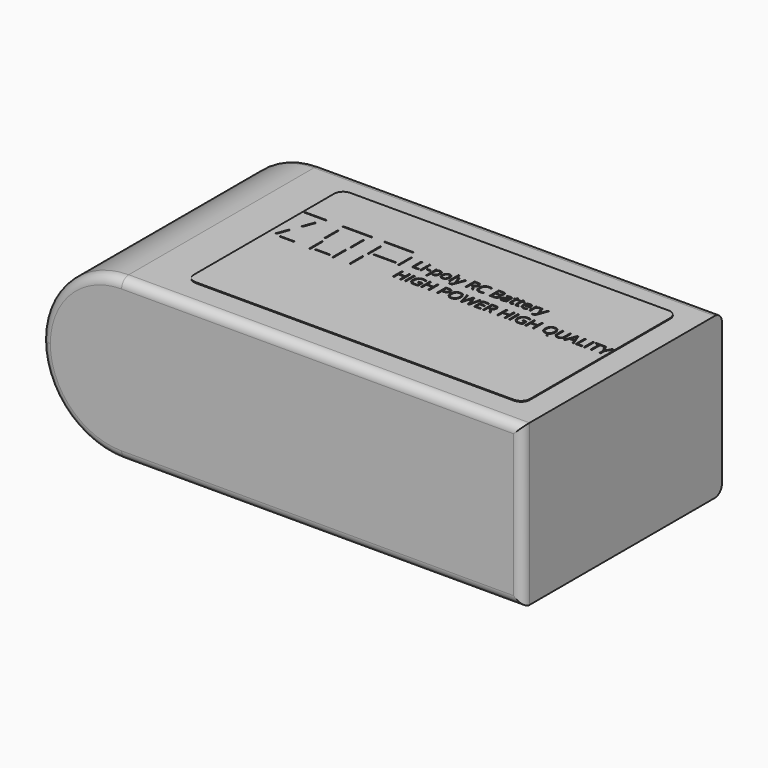
from build123d import *

# Parameters (mm, degrees)
F0_W     = 54
F0_H     = 28
F1_DEPTH = 18
F2_R     = 8.99999
F3_W     = 0.1241319444
F3_H     = 1.8092230903
F3_W_2   = 0.1498046875
F3_H_2   = 1.2889973958
F3_W_3   = 0.1464192708
F3_H_3   = 0.9662543403
F3_W_4   = 0.4327690972
F3_H_4   = 0.1340060764
F3_H_5   = 1.3719401042
F4_DEPTH = 0.1
F5_R     = 1


# Not quite as in the source:
# - a fillet or chamfer is up to 0.001 mm smaller than in the source, because OpenCascade refuses the exact size


with BuildPart() as f1:
    # F0 (on Top) → F1 (new body)
    with BuildSketch(Plane.XY):
        with Locations((-3.3961925656, 5.444671735)):
            Rectangle(F0_W, F0_H)
    extrude(amount=F1_DEPTH)

    # F2 (radius 9 in the source; OpenCascade refuses exactly that, so slightly less here)
    f2_edges = [f1.edges().sort_by_distance(p)[0] for p in [
        (-30.396193, 5.444672, 18),
        (-30.396193, 5.444672, 0),
    ]]
    fillet(f2_edges, radius=F2_R)

    # F3 (on face) → F4 (join)
    with BuildSketch(Plane.XY.offset(18)):
        with BuildLine():
            Line((19.9144558758, 16.5669198185), (-15.8251227587, 16.5669198185))
            ThreePointArc((-15.8251227587, 16.5669198185), (-16.5322295399, 16.2740265997), (-16.8251227587, 15.5669198185))
            Line((-16.8251227587, 15.5669198185), (-16.8251227587, -4.1303987275))
            ThreePointArc((-16.8251227587, -4.1303987275), (-16.5322295399, -4.8375055087), (-15.8251227587, -5.1303987275))
            Line((-15.8251227587, -5.1303987275), (19.9144558758, -5.1303987275))
            ThreePointArc((19.9144558758, -5.1303987275), (20.6215626569, -4.8375055087), (20.9144558758, -4.1303987275))
            Line((20.9144558758, -4.1303987275), (20.9144558758, 15.5669198185))
            ThreePointArc((20.9144558758, 15.5669198185), (20.6215626569, 16.2740265997), (19.9144558758, 16.5669198185))
        make_face()
        Polygon((-15.6610215548, 7.7806734869), (-15.514884402, 7.7806734869), (-15.9953314506, 6.4916760911), (-16.1414686034, 6.4916760911), align=None, mode=Mode.SUBTRACT)
        Polygon((-13.8740857909, 6.2140719244), (-14.6834824923, 6.2140719244), (-14.6905354437, 6.2140719244), (-15.4999321451, 6.2140719244), (-15.4999321451, 6.3294582091), (-14.6905354437, 6.3294582091), (-14.6834824923, 6.3294582091), (-13.8740857909, 6.3294582091), align=None, mode=Mode.SUBTRACT)
        Polygon((-9.8533392631, 6.2140719244), (-10.6627359645, 6.2140719244), (-10.6697889159, 6.2140719244), (-11.4791856173, 6.2140719244), (-11.4791856173, 6.3294582091), (-10.6697889159, 6.3294582091), (-10.6627359645, 6.3294582091), (-9.8533392631, 6.3294582091), align=None, mode=Mode.SUBTRACT)
        with Locations((-11.9723279784, 6.9590046501)):
            Rectangle(F3_W, F3_H, mode=Mode.SUBTRACT)
        Polygon((-14.722696902, 10.2362290425), (-14.5765597492, 10.2362290425), (-15.0570067979, 8.9472316466), (-15.2031439506, 8.9472316466), align=None, mode=Mode.SUBTRACT)
        with Locations((-12.183634402, 9.4145602057)):
            Rectangle(F3_W, F3_H, mode=Mode.SUBTRACT)
        Polygon((-15.0132784992, 11.1251830355), (-15.8156222492, 11.1251830355), (-15.8226752006, 11.1251830355), (-16.632071902, 11.1251830355), (-16.632071902, 11.2405693202), (-15.8226752006, 11.2405693202), (-15.8156222492, 11.2405693202), (-15.0132784992, 11.2405693202), (-15.0062255479, 11.2405693202), (-14.1968288465, 11.2405693202), (-14.1968288465, 11.1251830355), (-15.0062255479, 11.1251830355), align=None, mode=Mode.SUBTRACT)
        Polygon((-10.7084390895, 11.1251830355), (-11.5107828395, 11.1251830355), (-11.5178357909, 11.1251830355), (-12.3272324923, 11.1251830355), (-12.3272324923, 11.2405693202), (-11.5178357909, 11.2405693202), (-11.5107828395, 11.2405693202), (-10.7084390895, 11.2405693202), (-10.7013861381, 11.2405693202), (-9.8990423881, 11.2405693202), (-9.8919894367, 11.2405693202), (-9.0825927354, 11.2405693202), (-9.0825927354, 11.1251830355), (-9.8919894367, 11.1251830355), (-9.8990423881, 11.1251830355), (-10.7013861381, 11.1251830355), align=None, mode=Mode.SUBTRACT)
        with Locations((-9.3590684298, 6.9590046501)):
            Rectangle(F3_W, F3_H, mode=Mode.SUBTRACT)
        with Locations((-7.4262776312, 6.9590046501)):
            Rectangle(F3_W, F3_H, mode=Mode.SUBTRACT)
        Polygon((-5.2677923881, 8.66962748), (-6.0701361381, 8.66962748), (-6.0771890895, 8.66962748), (-6.8865857909, 8.66962748), (-6.8865857909, 8.7850137647), (-6.0771890895, 8.7850137647), (-6.0701361381, 8.7850137647), (-5.2677923881, 8.7850137647), (-5.2607394367, 8.7850137647), (-4.4513427354, 8.7850137647), (-4.4513427354, 8.66962748), (-5.2607394367, 8.66962748), align=None, mode=Mode.SUBTRACT)
        Polygon((-2.0203314506, 7.7806734869), (-2.0203314506, 6.4916760911), (-2.1701361381, 6.4916760911), (-2.1701361381, 7.0982299105), (-2.8491942979, 7.0982299105), (-2.8491942979, 6.4916760911), (-2.9989989854, 6.4916760911), (-2.9989989854, 7.7806734869), (-2.8491942979, 7.7806734869), (-2.8491942979, 7.2322359869), (-2.1701361381, 7.2322359869), (-2.1701361381, 7.7806734869), align=None, mode=Mode.SUBTRACT)
        with Locations((-1.5919351833, 7.136174789)):
            Rectangle(F3_W_2, F3_H_2, mode=Mode.SUBTRACT)
        with BuildLine():
            Line((-0.5964816242, 7.0330606397), (-0.5964816242, 7.1670667161))
            Line((-0.5964816242, 7.1670667161), (-0.158352284, 7.1670667161))
            Line((-0.158352284, 7.1670667161), (-0.158352284, 6.5402003966))
            add(Edge.make_bspline(
                [(-0.158352284, 6.5402003966), (-0.2607611381, 6.5074747022), (-0.366555409, 6.4906886779)],
                knots=[0, 0, 0, 1, 1, 1], degree=2))
            add(Edge.make_bspline(
                [(-0.366555409, 6.4906886779), (-0.4723496798, 6.4739026536), (-0.6117159992, 6.4739026536)],
                knots=[0, 0, 0, 1, 1, 1], degree=2))
            add(Edge.make_bspline(
                [(-0.6117159992, 6.4739026536), (-0.9042724229, 6.4739026536), (-1.067336659, 6.6481105529)],
                knots=[0, 0, 0, 1, 1, 1], degree=2))
            add(Edge.make_bspline(
                [(-1.067336659, 6.6481105529), (-1.2304008951, 6.8223184522), (-1.2304008951, 7.13603373)],
                knots=[0, 0, 0, 1, 1, 1], degree=2))
            add(Edge.make_bspline(
                [(-1.2304008951, 7.13603373), (-1.2304008951, 7.3371839036), (-1.1497151312, 7.4883991813)],
                knots=[0, 0, 0, 1, 1, 1], degree=2))
            add(Edge.make_bspline(
                [(-1.1497151312, 7.4883991813), (-1.0690293673, 7.6396144591), (-0.9173909124, 7.7193128098)],
                knots=[0, 0, 0, 1, 1, 1], degree=2))
            add(Edge.make_bspline(
                [(-0.9173909124, 7.7193128098), (-0.7657524576, 7.7990111605), (-0.5623453395, 7.7990111605)],
                knots=[0, 0, 0, 1, 1, 1], degree=2))
            add(Edge.make_bspline(
                [(-0.5623453395, 7.7990111605), (-0.3558349229, 7.7990111605), (-0.1778184298, 7.7234035216)],
                knots=[0, 0, 0, 1, 1, 1], degree=2))
            Line((-0.1778184298, 7.7234035216), (-0.2359347492, 7.5910901536))
            add(Edge.make_bspline(
                [(-0.2359347492, 7.5910901536), (-0.4105658256, 7.6650050841), (-0.5719373534, 7.6650050841)],
                knots=[0, 0, 0, 1, 1, 1], degree=2))
            add(Edge.make_bspline(
                [(-0.5719373534, 7.6650050841), (-0.8072238117, 7.6650050841), (-0.9395371798, 7.5249334695)],
                knots=[0, 0, 0, 1, 1, 1], degree=2))
            add(Edge.make_bspline(
                [(-0.9395371798, 7.5249334695), (-1.0718505479, 7.384861855), (-1.0718505479, 7.13603373)],
                knots=[0, 0, 0, 1, 1, 1], degree=2))
            add(Edge.make_bspline(
                [(-1.0718505479, 7.13603373), (-1.0718505479, 6.8750745286), (-0.9444742458, 6.740222098)],
                knots=[0, 0, 0, 1, 1, 1], degree=2))
            add(Edge.make_bspline(
                [(-0.9444742458, 6.740222098), (-0.8170979437, 6.6053696675), (-0.5702446451, 6.6053696675)],
                knots=[0, 0, 0, 1, 1, 1], degree=2))
            add(Edge.make_bspline(
                [(-0.5702446451, 6.6053696675), (-0.4362385687, 6.6053696675), (-0.3084390895, 6.6364026536)],
                knots=[0, 0, 0, 1, 1, 1], degree=2))
            Line((-0.3084390895, 6.6364026536), (-0.3084390895, 7.0330606397))
            Line((-0.3084390895, 7.0330606397), (-0.5964816242, 7.0330606397))
        make_face(mode=Mode.SUBTRACT)
        Polygon((1.1295166396, 7.7806734869), (1.1295166396, 6.4916760911), (0.9797119521, 6.4916760911), (0.9797119521, 7.0982299105), (0.3006537924, 7.0982299105), (0.3006537924, 6.4916760911), (0.1508491049, 6.4916760911), (0.1508491049, 7.7806734869), (0.3006537924, 7.7806734869), (0.3006537924, 7.2322359869), (0.9797119521, 7.2322359869), (0.9797119521, 7.7806734869), align=None, mode=Mode.SUBTRACT)
        with Locations((-9.3125189506, 9.4145602057)):
            Rectangle(F3_W, F3_H, mode=Mode.SUBTRACT)
        with Locations((-7.379728152, 9.4145602057)):
            Rectangle(F3_W, F3_H, mode=Mode.SUBTRACT)
        Polygon((-6.0633653048, 11.1251830355), (-6.8657090548, 11.1251830355), (-6.8727620062, 11.1251830355), (-7.6821587076, 11.1251830355), (-7.6821587076, 11.2405693202), (-6.8727620062, 11.2405693202), (-6.8657090548, 11.2405693202), (-6.0633653048, 11.2405693202), (-6.0563123534, 11.2405693202), (-5.2539686034, 11.2405693202), (-5.246915652, 11.2405693202), (-4.4375189506, 11.2405693202), (-4.4375189506, 11.1251830355), (-5.246915652, 11.1251830355), (-5.2539686034, 11.1251830355), (-6.0563123534, 11.1251830355), align=None, mode=Mode.SUBTRACT)
        with Locations((-3.957071902, 9.4145602057)):
            Rectangle(F3_W, F3_H, mode=Mode.SUBTRACT)
        Polygon((-2.0953748534, 8.9472316466), (-2.8139295409, 8.9472316466), (-2.8139295409, 10.2362290425), (-2.6641248534, 10.2362290425), (-2.6641248534, 9.0829304313), (-2.0953748534, 9.0829304313), align=None, mode=Mode.SUBTRACT)
        with Locations((-1.8255289333, 9.4303588168)):
            Rectangle(F3_W_3, F3_H_3, mode=Mode.SUBTRACT)
        with BuildLine():
            add(Edge.make_bspline(
                [(-1.8864664333, 10.10165873), (-1.9111517631, 10.1259208827), (-1.9111517631, 10.1752915425)],
                knots=[0, 0, 0, 1, 1, 1], degree=2))
            add(Edge.make_bspline(
                [(-1.9111517631, 10.1752915425), (-1.9111517631, 10.2255085563), (-1.8864664333, 10.248924355)],
                knots=[0, 0, 0, 1, 1, 1], degree=2))
            add(Edge.make_bspline(
                [(-1.8864664333, 10.248924355), (-1.8617811034, 10.2723401536), (-1.8245415201, 10.2723401536)],
                knots=[0, 0, 0, 1, 1, 1], degree=2))
            add(Edge.make_bspline(
                [(-1.8245415201, 10.2723401536), (-1.7892767631, 10.2723401536), (-1.7637450791, 10.2485011779)],
                knots=[0, 0, 0, 1, 1, 1], degree=2))
            add(Edge.make_bspline(
                [(-1.7637450791, 10.2485011779), (-1.7382133951, 10.2246622022), (-1.7382133951, 10.1752915425)],
                knots=[0, 0, 0, 1, 1, 1], degree=2))
            add(Edge.make_bspline(
                [(-1.7382133951, 10.1752915425), (-1.7382133951, 10.1259208827), (-1.7637450791, 10.10165873)],
                knots=[0, 0, 0, 1, 1, 1], degree=2))
            add(Edge.make_bspline(
                [(-1.7637450791, 10.10165873), (-1.7892767631, 10.0773965772), (-1.8245415201, 10.0773965772)],
                knots=[0, 0, 0, 1, 1, 1], degree=2))
            add(Edge.make_bspline(
                [(-1.8245415201, 10.0773965772), (-1.8617811034, 10.0773965772), (-1.8864664333, 10.10165873)],
                knots=[0, 0, 0, 1, 1, 1], degree=2))
        make_face(mode=Mode.SUBTRACT)
        with BuildLine():
            add(Edge.make_bspline(
                [(-0.1164577527, 9.0613484001), (-0.2226752006, 8.9294582091), (-0.4114121798, 8.9294582091)],
                knots=[0, 0, 0, 1, 1, 1], degree=2))
            add(Edge.make_bspline(
                [(-0.4114121798, 8.9294582091), (-0.5059217284, 8.9294582091), (-0.5839273708, 8.964299789)],
                knots=[0, 0, 0, 1, 1, 1], degree=2))
            add(Edge.make_bspline(
                [(-0.5839273708, 8.964299789), (-0.6619330131, 8.9991413688), (-0.7146890895, 9.0716457091)],
                knots=[0, 0, 0, 1, 1, 1], degree=2))
            Line((-0.7146890895, 9.0716457091), (-0.7254095756, 9.0716457091))
            add(Edge.make_bspline(
                [(-0.7254095756, 9.0716457091), (-0.7146890895, 8.9870102925), (-0.7146890895, 8.9111205355)],
                knots=[0, 0, 0, 1, 1, 1], degree=2))
            Line((-0.7146890895, 8.9111205355), (-0.7146890895, 8.5133340772))
            Line((-0.7146890895, 8.5133340772), (-0.8611083604, 8.5133340772))
            Line((-0.8611083604, 8.5133340772), (-0.8611083604, 9.9134859869))
            Line((-0.8611083604, 9.9134859869), (-0.7420545409, 9.9134859869))
            Line((-0.7420545409, 9.9134859869), (-0.7217420409, 9.7811726188))
            Line((-0.7217420409, 9.7811726188), (-0.7146890895, 9.7811726188))
            add(Edge.make_bspline(
                [(-0.7146890895, 9.7811726188), (-0.6582654784, 9.8607299105), (-0.5833631347, 9.8959946675)],
                knots=[0, 0, 0, 1, 1, 1], degree=2))
            add(Edge.make_bspline(
                [(-0.5833631347, 9.8959946675), (-0.5084607909, 9.9312594244), (-0.4114121798, 9.9312594244)],
                knots=[0, 0, 0, 1, 1, 1], degree=2))
            add(Edge.make_bspline(
                [(-0.4114121798, 9.9312594244), (-0.219289784, 9.9312594244), (-0.1147650444, 9.7997924105)],
                knots=[0, 0, 0, 1, 1, 1], degree=2))
            add(Edge.make_bspline(
                [(-0.1147650444, 9.7997924105), (-0.0102403048, 9.6683253966), (-0.0102403048, 9.43134623)],
                knots=[0, 0, 0, 1, 1, 1], degree=2))
            add(Edge.make_bspline(
                [(-0.0102403048, 9.43134623), (-0.0102403048, 9.1932385911), (-0.1164577527, 9.0613484001)],
                knots=[0, 0, 0, 1, 1, 1], degree=2))
        make_face(mode=Mode.SUBTRACT)
        with Locations((-1.3065727701, 9.4312051709)):
            Rectangle(F3_W_4, F3_H_4, mode=Mode.SUBTRACT)
        with BuildLine():
            add(Edge.make_bspline(
                [(0.9598226292, 9.7962659348), (1.0792996258, 9.6612724452), (1.0792996258, 9.43134623)],
                knots=[0, 0, 0, 1, 1, 1], degree=2))
            add(Edge.make_bspline(
                [(1.0792996258, 9.43134623), (1.0792996258, 9.1949312994), (0.9603868653, 9.0621947543)],
                knots=[0, 0, 0, 1, 1, 1], degree=2))
            add(Edge.make_bspline(
                [(0.9603868653, 9.0621947543), (0.8414741049, 8.9294582091), (0.6315782716, 8.9294582091)],
                knots=[0, 0, 0, 1, 1, 1], degree=2))
            add(Edge.make_bspline(
                [(0.6315782716, 8.9294582091), (0.501803966, 8.9294582091), (0.4013699383, 8.9903957091)],
                knots=[0, 0, 0, 1, 1, 1], degree=2))
            add(Edge.make_bspline(
                [(0.4013699383, 8.9903957091), (0.3009359105, 9.0513332091), (0.2462050077, 9.1650267855)],
                knots=[0, 0, 0, 1, 1, 1], degree=2))
            add(Edge.make_bspline(
                [(0.2462050077, 9.1650267855), (0.1914741049, 9.2787203619), (0.1914741049, 9.43134623)],
                knots=[0, 0, 0, 1, 1, 1], degree=2))
            add(Edge.make_bspline(
                [(0.1914741049, 9.43134623), (0.1914741049, 9.6674790425), (0.3096815702, 9.7993692334)],
                knots=[0, 0, 0, 1, 1, 1], degree=2))
            add(Edge.make_bspline(
                [(0.3096815702, 9.7993692334), (0.4278890355, 9.9312594244), (0.6377848688, 9.9312594244)],
                knots=[0, 0, 0, 1, 1, 1], degree=2))
            add(Edge.make_bspline(
                [(0.6377848688, 9.9312594244), (0.8403456327, 9.9312594244), (0.9598226292, 9.7962659348)],
                knots=[0, 0, 0, 1, 1, 1], degree=2))
        make_face(mode=Mode.SUBTRACT)
        with BuildLine():
            add(Edge.make_bspline(
                [(2.2864827855, 7.7806734869), (2.7694688966, 7.7806734869), (2.7694688966, 7.405174355)],
                knots=[0, 0, 0, 1, 1, 1], degree=2))
            add(Edge.make_bspline(
                [(2.7694688966, 7.405174355), (2.7694688966, 7.2093844244), (2.6358859973, 7.1040133307)],
                knots=[0, 0, 0, 1, 1, 1], degree=2))
            add(Edge.make_bspline(
                [(2.6358859973, 7.1040133307), (2.502303098, 6.9986422369), (2.253757091, 6.9986422369)],
                knots=[0, 0, 0, 1, 1, 1], degree=2))
            Line((2.253757091, 6.9986422369), (2.1019775771, 6.9986422369))
            Line((2.1019775771, 6.9986422369), (2.1019775771, 6.4916760911))
            Line((2.1019775771, 6.4916760911), (1.9521728896, 6.4916760911))
            Line((1.9521728896, 6.4916760911), (1.9521728896, 7.7806734869))
            Line((1.9521728896, 7.7806734869), (2.2864827855, 7.7806734869))
        make_face(mode=Mode.SUBTRACT)
        with BuildLine():
            add(Edge.make_bspline(
                [(4.0020426813, 7.6246622022), (4.158053966, 7.4483384175), (4.158053966, 7.1380085563)],
                knots=[0, 0, 0, 1, 1, 1], degree=2))
            add(Edge.make_bspline(
                [(4.158053966, 7.1380085563), (4.158053966, 6.8285250494), (4.0014784452, 6.6512138515)],
                knots=[0, 0, 0, 1, 1, 1], degree=2))
            add(Edge.make_bspline(
                [(4.0014784452, 6.6512138515), (3.8449029244, 6.4739026536), (3.5664524035, 6.4739026536)],
                knots=[0, 0, 0, 1, 1, 1], degree=2))
            add(Edge.make_bspline(
                [(3.5664524035, 6.4739026536), (3.2817952855, 6.4739026536), (3.127053532, 6.6481105529)],
                knots=[0, 0, 0, 1, 1, 1], degree=2))
            add(Edge.make_bspline(
                [(3.127053532, 6.6481105529), (2.9723117785, 6.8223184522), (2.9723117785, 7.1397012647)],
                knots=[0, 0, 0, 1, 1, 1], degree=2))
            add(Edge.make_bspline(
                [(2.9723117785, 7.1397012647), (2.9723117785, 7.4545450147), (3.1274767091, 7.6277655008)],
                knots=[0, 0, 0, 1, 1, 1], degree=2))
            add(Edge.make_bspline(
                [(3.1274767091, 7.6277655008), (3.2826416396, 7.8009859869), (3.5681451119, 7.8009859869)],
                knots=[0, 0, 0, 1, 1, 1], degree=2))
            add(Edge.make_bspline(
                [(3.5681451119, 7.8009859869), (3.8460313966, 7.8009859869), (4.0020426813, 7.6246622022)],
                knots=[0, 0, 0, 1, 1, 1], degree=2))
        make_face(mode=Mode.SUBTRACT)
        with BuildLine():
            Line((5.915085216, 7.7806734869), (5.5703369521, 6.4916760911))
            Line((5.5703369521, 6.4916760911), (5.422224973, 6.4916760911))
            Line((5.422224973, 6.4916760911), (5.1621121258, 7.354675223))
            add(Edge.make_bspline(
                [(5.1621121258, 7.354675223), (5.1434923341, 7.4122273063), (5.1206407716, 7.4994017855)],
                knots=[0, 0, 0, 1, 1, 1], degree=2))
            add(Edge.make_bspline(
                [(5.1206407716, 7.4994017855), (5.0977892091, 7.5865762647), (5.0969428549, 7.6043497022)],
                knots=[0, 0, 0, 1, 1, 1], degree=2))
            add(Edge.make_bspline(
                [(5.0969428549, 7.6043497022), (5.0774767091, 7.4878349452), (5.0351590008, 7.349597098)],
                knots=[0, 0, 0, 1, 1, 1], degree=2))
            Line((5.0351590008, 7.349597098), (4.7829454591, 6.4916760911))
            Line((4.7829454591, 6.4916760911), (4.6348334799, 6.4916760911))
            Line((4.6348334799, 6.4916760911), (4.2917779244, 7.7806734869))
            Line((4.2917779244, 7.7806734869), (4.4506103896, 7.7806734869))
            Line((4.4506103896, 7.7806734869), (4.6542996258, 6.9845363341))
            add(Edge.make_bspline(
                [(4.6542996258, 6.9845363341), (4.6966173341, 6.8169582091), (4.7160834799, 6.6812594244)],
                knots=[0, 0, 0, 1, 1, 1], degree=2))
            add(Edge.make_bspline(
                [(4.7160834799, 6.6812594244), (4.7397813966, 6.8426309522), (4.7866129938, 6.9969495286)],
                knots=[0, 0, 0, 1, 1, 1], degree=2))
            Line((4.7866129938, 6.9969495286), (5.0173855633, 7.7806734869))
            Line((5.0173855633, 7.7806734869), (5.1762180285, 7.7806734869))
            Line((5.1762180285, 7.7806734869), (5.4185574383, 6.9898965772))
            add(Edge.make_bspline(
                [(5.4185574383, 6.9898965772), (5.4608751466, 6.8530693202), (5.4899333063, 6.6812594244)],
                knots=[0, 0, 0, 1, 1, 1], degree=2))
            add(Edge.make_bspline(
                [(5.4899333063, 6.6812594244), (5.5068603896, 6.8065198411), (5.5534098688, 6.9862290425)],
                knots=[0, 0, 0, 1, 1, 1], degree=2))
            Line((5.5534098688, 6.9862290425), (5.7562527508, 7.7806734869))
            Line((5.7562527508, 7.7806734869), (5.915085216, 7.7806734869))
        make_face(mode=Mode.SUBTRACT)
        Polygon((6.8353543133, 6.6256821675), (6.8353543133, 6.4916760911), (6.1167996258, 6.4916760911), (6.1167996258, 7.7806734869), (6.8353543133, 7.7806734869), (6.8353543133, 7.6475137647), (6.2666043133, 7.6475137647), (6.2666043133, 7.2322359869), (6.8009359105, 7.2322359869), (6.8009359105, 7.0999226188), (6.2666043133, 7.0999226188), (6.2666043133, 6.6256821675), align=None, mode=Mode.SUBTRACT)
        with BuildLine():
            Line((7.539803098, 7.0277003966), (7.270662473, 7.0277003966))
            Line((7.270662473, 7.0277003966), (7.270662473, 6.4916760911))
            Line((7.270662473, 6.4916760911), (7.1208577855, 6.4916760911))
            Line((7.1208577855, 6.4916760911), (7.1208577855, 7.7806734869))
            Line((7.1208577855, 7.7806734869), (7.4743517091, 7.7806734869))
            add(Edge.make_bspline(
                [(7.4743517091, 7.7806734869), (7.7116129938, 7.7806734869), (7.8248833931, 7.689831473)],
                knots=[0, 0, 0, 1, 1, 1], degree=2))
            add(Edge.make_bspline(
                [(7.8248833931, 7.689831473), (7.9381537924, 7.5989894591), (7.9381537924, 7.4164590772)],
                knots=[0, 0, 0, 1, 1, 1], degree=2))
            add(Edge.make_bspline(
                [(7.9381537924, 7.4164590772), (7.9381537924, 7.1608601188), (7.6788872994, 7.0708644591)],
                knots=[0, 0, 0, 1, 1, 1], degree=2))
            Line((7.6788872994, 7.0708644591), (8.0289958063, 6.4916760911))
            Line((8.0289958063, 6.4916760911), (7.8518256674, 6.4916760911))
            Line((7.8518256674, 6.4916760911), (7.539803098, 7.0277003966))
        make_face(mode=Mode.SUBTRACT)
        Polygon((9.6847466744, 7.7806734869), (9.6847466744, 6.4916760911), (9.5349419869, 6.4916760911), (9.5349419869, 7.0982299105), (8.8558838271, 7.0982299105), (8.8558838271, 6.4916760911), (8.7060791396, 6.4916760911), (8.7060791396, 7.7806734869), (8.8558838271, 7.7806734869), (8.8558838271, 7.2322359869), (9.5349419869, 7.2322359869), (9.5349419869, 7.7806734869), align=None, mode=Mode.SUBTRACT)
        with Locations((10.1131429417, 7.136174789)):
            Rectangle(F3_W_2, F3_H_2, mode=Mode.SUBTRACT)
        with BuildLine():
            Line((11.1085965008, 7.0330606397), (11.1085965008, 7.1670667161))
            Line((11.1085965008, 7.1670667161), (11.546725841, 7.1670667161))
            Line((11.546725841, 7.1670667161), (11.546725841, 6.5402003966))
            add(Edge.make_bspline(
                [(11.546725841, 6.5402003966), (11.4443169869, 6.5074747022), (11.338522716, 6.4906886779)],
                knots=[0, 0, 0, 1, 1, 1], degree=2))
            add(Edge.make_bspline(
                [(11.338522716, 6.4906886779), (11.2327284452, 6.4739026536), (11.0933621258, 6.4739026536)],
                knots=[0, 0, 0, 1, 1, 1], degree=2))
            add(Edge.make_bspline(
                [(11.0933621258, 6.4739026536), (10.8008057021, 6.4739026536), (10.637741466, 6.6481105529)],
                knots=[0, 0, 0, 1, 1, 1], degree=2))
            add(Edge.make_bspline(
                [(10.637741466, 6.6481105529), (10.4746772299, 6.8223184522), (10.4746772299, 7.13603373)],
                knots=[0, 0, 0, 1, 1, 1], degree=2))
            add(Edge.make_bspline(
                [(10.4746772299, 7.13603373), (10.4746772299, 7.3371839036), (10.5553629938, 7.4883991813)],
                knots=[0, 0, 0, 1, 1, 1], degree=2))
            add(Edge.make_bspline(
                [(10.5553629938, 7.4883991813), (10.6360487577, 7.6396144591), (10.7876872126, 7.7193128098)],
                knots=[0, 0, 0, 1, 1, 1], degree=2))
            add(Edge.make_bspline(
                [(10.7876872126, 7.7193128098), (10.9393256674, 7.7990111605), (11.1427327855, 7.7990111605)],
                knots=[0, 0, 0, 1, 1, 1], degree=2))
            add(Edge.make_bspline(
                [(11.1427327855, 7.7990111605), (11.3492432021, 7.7990111605), (11.5272596952, 7.7234035216)],
                knots=[0, 0, 0, 1, 1, 1], degree=2))
            Line((11.5272596952, 7.7234035216), (11.4691433758, 7.5910901536))
            add(Edge.make_bspline(
                [(11.4691433758, 7.5910901536), (11.2945122994, 7.6650050841), (11.1331407716, 7.6650050841)],
                knots=[0, 0, 0, 1, 1, 1], degree=2))
            add(Edge.make_bspline(
                [(11.1331407716, 7.6650050841), (10.8978543133, 7.6650050841), (10.7655409452, 7.5249334695)],
                knots=[0, 0, 0, 1, 1, 1], degree=2))
            add(Edge.make_bspline(
                [(10.7655409452, 7.5249334695), (10.6332275771, 7.384861855), (10.6332275771, 7.13603373)],
                knots=[0, 0, 0, 1, 1, 1], degree=2))
            add(Edge.make_bspline(
                [(10.6332275771, 7.13603373), (10.6332275771, 6.8750745286), (10.7606038792, 6.740222098)],
                knots=[0, 0, 0, 1, 1, 1], degree=2))
            add(Edge.make_bspline(
                [(10.7606038792, 6.740222098), (10.8879801813, 6.6053696675), (11.1348334799, 6.6053696675)],
                knots=[0, 0, 0, 1, 1, 1], degree=2))
            add(Edge.make_bspline(
                [(11.1348334799, 6.6053696675), (11.2688395563, 6.6053696675), (11.3966390355, 6.6364026536)],
                knots=[0, 0, 0, 1, 1, 1], degree=2))
            Line((11.3966390355, 6.6364026536), (11.3966390355, 7.0330606397))
            Line((11.3966390355, 7.0330606397), (11.1085965008, 7.0330606397))
        make_face(mode=Mode.SUBTRACT)
        Polygon((12.8345947646, 7.7806734869), (12.8345947646, 6.4916760911), (12.6847900771, 6.4916760911), (12.6847900771, 7.0982299105), (12.0057319174, 7.0982299105), (12.0057319174, 6.4916760911), (11.8559272299, 6.4916760911), (11.8559272299, 7.7806734869), (12.0057319174, 7.7806734869), (12.0057319174, 7.2322359869), (12.6847900771, 7.2322359869), (12.6847900771, 7.7806734869), align=None, mode=Mode.SUBTRACT)
        with BuildLine():
            Line((2.0291911188, 8.9418714036), (1.639303966, 9.9134859869))
            Line((1.639303966, 9.9134859869), (1.796443723, 9.9134859869))
            Line((1.796443723, 9.9134859869), (2.0080322646, 9.3625094244))
            add(Edge.make_bspline(
                [(2.0080322646, 9.3625094244), (2.0774333063, 9.1737724452), (2.0943603896, 9.0899833827)],
                knots=[0, 0, 0, 1, 1, 1], degree=2))
            Line((2.0943603896, 9.0899833827), (2.101413341, 9.0899833827))
            add(Edge.make_bspline(
                [(2.101413341, 9.0899833827), (2.1126980633, 9.1351222716), (2.1493734105, 9.2440198411)],
                knots=[0, 0, 0, 1, 1, 1], degree=2))
            add(Edge.make_bspline(
                [(2.1493734105, 9.2440198411), (2.1860487577, 9.3529174105), (2.3888916396, 9.9134859869)],
                knots=[0, 0, 0, 1, 1, 1], degree=2))
            Line((2.3888916396, 9.9134859869), (2.5457492785, 9.9134859869))
            Line((2.5457492785, 9.9134859869), (2.1304715008, 8.8132255702))
            add(Edge.make_bspline(
                [(2.1304715008, 8.8132255702), (2.0686876466, 8.6501613341), (1.9863091744, 8.5817477057)],
                knots=[0, 0, 0, 1, 1, 1], degree=2))
            add(Edge.make_bspline(
                [(1.9863091744, 8.5817477057), (1.9039307021, 8.5133340772), (1.7840305285, 8.5133340772)],
                knots=[0, 0, 0, 1, 1, 1], degree=2))
            add(Edge.make_bspline(
                [(1.7840305285, 8.5133340772), (1.7168864313, 8.5133340772), (1.6517171605, 8.5285684522)],
                knots=[0, 0, 0, 1, 1, 1], degree=2))
            Line((1.6517171605, 8.5285684522), (1.6517171605, 8.6456474452))
            add(Edge.make_bspline(
                [(1.6517171605, 8.6456474452), (1.700241466, 8.6352090772), (1.7600504938, 8.6352090772)],
                knots=[0, 0, 0, 1, 1, 1], degree=2))
            add(Edge.make_bspline(
                [(1.7600504938, 8.6352090772), (1.9109836535, 8.6352090772), (1.9753065702, 8.8044799105)],
                knots=[0, 0, 0, 1, 1, 1], degree=2))
            Line((1.9753065702, 8.8044799105), (2.0291911188, 8.9418714036))
        make_face(mode=Mode.SUBTRACT)
        with Locations((1.4092366917, 9.6332016987)):
            Rectangle(F3_W_3, F3_H_5, mode=Mode.SUBTRACT)
        with BuildLine():
            Line((3.6127197646, 9.4832559522), (3.3435791396, 9.4832559522))
            Line((3.3435791396, 9.4832559522), (3.3435791396, 8.9472316466))
            Line((3.3435791396, 8.9472316466), (3.1937744521, 8.9472316466))
            Line((3.1937744521, 8.9472316466), (3.1937744521, 10.2362290425))
            Line((3.1937744521, 10.2362290425), (3.5472683758, 10.2362290425))
            add(Edge.make_bspline(
                [(3.5472683758, 10.2362290425), (3.7845296605, 10.2362290425), (3.8978000598, 10.1453870286)],
                knots=[0, 0, 0, 1, 1, 1], degree=2))
            add(Edge.make_bspline(
                [(3.8978000598, 10.1453870286), (4.0110704591, 10.0545450147), (4.0110704591, 9.8720146327)],
                knots=[0, 0, 0, 1, 1, 1], degree=2))
            add(Edge.make_bspline(
                [(4.0110704591, 9.8720146327), (4.0110704591, 9.6164156744), (3.751803966, 9.5264200147)],
                knots=[0, 0, 0, 1, 1, 1], degree=2))
            Line((3.751803966, 9.5264200147), (4.101912473, 8.9472316466))
            Line((4.101912473, 8.9472316466), (3.9247423341, 8.9472316466))
            Line((3.9247423341, 8.9472316466), (3.6127197646, 9.4832559522))
        make_face(mode=Mode.SUBTRACT)
        with BuildLine():
            add(Edge.make_bspline(
                [(5.1544949383, 10.0520059522), (5.0080756674, 10.1205606397), (4.8616563966, 10.1205606397)],
                knots=[0, 0, 0, 1, 1, 1], degree=2))
            add(Edge.make_bspline(
                [(4.8616563966, 10.1205606397), (4.6492215008, 10.1205606397), (4.5262180285, 9.9790784348)],
                knots=[0, 0, 0, 1, 1, 1], degree=2))
            add(Edge.make_bspline(
                [(4.5262180285, 9.9790784348), (4.4032145563, 9.83759623), (4.4032145563, 9.5915892855)],
                knots=[0, 0, 0, 1, 1, 1], degree=2))
            add(Edge.make_bspline(
                [(4.4032145563, 9.5915892855), (4.4032145563, 9.3388115077), (4.5218451987, 9.2007147195)],
                knots=[0, 0, 0, 1, 1, 1], degree=2))
            add(Edge.make_bspline(
                [(4.5218451987, 9.2007147195), (4.640475841, 9.0626179313), (4.8599636883, 9.0626179313)],
                knots=[0, 0, 0, 1, 1, 1], degree=2))
            add(Edge.make_bspline(
                [(4.8599636883, 9.0626179313), (4.9948161188, 9.0626179313), (5.1677544869, 9.1111422369)],
                knots=[0, 0, 0, 1, 1, 1], degree=2))
            Line((5.1677544869, 9.1111422369), (5.1677544869, 8.9799573411))
            add(Edge.make_bspline(
                [(5.1677544869, 8.9799573411), (5.0337484105, 8.9294582091), (4.8371121258, 8.9294582091)],
                knots=[0, 0, 0, 1, 1, 1], degree=2))
            add(Edge.make_bspline(
                [(4.8371121258, 8.9294582091), (4.5524550077, 8.9294582091), (4.3977132542, 9.1023965772)],
                knots=[0, 0, 0, 1, 1, 1], degree=2))
            add(Edge.make_bspline(
                [(4.3977132542, 9.1023965772), (4.2429715008, 9.2753349452), (4.2429715008, 9.5935641119)],
                knots=[0, 0, 0, 1, 1, 1], degree=2))
            add(Edge.make_bspline(
                [(4.2429715008, 9.5935641119), (4.2429715008, 9.7927394591), (4.3174506674, 9.9425441466)],
                knots=[0, 0, 0, 1, 1, 1], degree=2))
            add(Edge.make_bspline(
                [(4.3174506674, 9.9425441466), (4.3919298341, 10.0923488341), (4.5325656848, 10.1734577751)],
                knots=[0, 0, 0, 1, 1, 1], degree=2))
            add(Edge.make_bspline(
                [(4.5325656848, 10.1734577751), (4.6732015355, 10.2545667161), (4.863631223, 10.2545667161)],
                knots=[0, 0, 0, 1, 1, 1], degree=2))
            add(Edge.make_bspline(
                [(4.863631223, 10.2545667161), (5.0661919869, 10.2545667161), (5.2179715008, 10.1806517855)],
                knots=[0, 0, 0, 1, 1, 1], degree=2))
            Line((5.2179715008, 10.1806517855), (5.1544949383, 10.0520059522))
        make_face(mode=Mode.SUBTRACT)
        with BuildLine():
            Line((5.9181885146, 8.9472316466), (5.9181885146, 10.2362290425))
            Line((5.9181885146, 10.2362290425), (6.2824029244, 10.2362290425))
            add(Edge.make_bspline(
                [(6.2824029244, 10.2362290425), (6.5388482369, 10.2362290425), (6.6535292264, 10.1594929313)],
                knots=[0, 0, 0, 1, 1, 1], degree=2))
            add(Edge.make_bspline(
                [(6.6535292264, 10.1594929313), (6.768210216, 10.0827568202), (6.768210216, 9.9171535216)],
                knots=[0, 0, 0, 1, 1, 1], degree=2))
            add(Edge.make_bspline(
                [(6.768210216, 9.9171535216), (6.768210216, 9.802331473), (6.7043104764, 9.7278523063)],
                knots=[0, 0, 0, 1, 1, 1], degree=2))
            add(Edge.make_bspline(
                [(6.7043104764, 9.7278523063), (6.6404107369, 9.6533731397), (6.5176893827, 9.6313679313)],
                knots=[0, 0, 0, 1, 1, 1], degree=2))
            Line((6.5176893827, 9.6313679313), (6.5176893827, 9.6226222716))
            add(Edge.make_bspline(
                [(6.5176893827, 9.6226222716), (6.8113742785, 9.5724052577), (6.8113742785, 9.3139851188)],
                knots=[0, 0, 0, 1, 1, 1], degree=2))
            add(Edge.make_bspline(
                [(6.8113742785, 9.3139851188), (6.8113742785, 9.1413288688), (6.6945774035, 9.0442802577)],
                knots=[0, 0, 0, 1, 1, 1], degree=2))
            add(Edge.make_bspline(
                [(6.6945774035, 9.0442802577), (6.5777805285, 8.9472316466), (6.3678846952, 8.9472316466)],
                knots=[0, 0, 0, 1, 1, 1], degree=2))
            Line((6.3678846952, 8.9472316466), (5.9181885146, 8.9472316466))
        make_face(mode=Mode.SUBTRACT)
        with BuildLine():
            Line((7.7688829591, 8.9472316466), (7.6602675077, 8.9472316466))
            Line((7.6602675077, 8.9472316466), (7.631209348, 9.0849052577))
            Line((7.631209348, 9.0849052577), (7.6241563966, 9.0849052577))
            add(Edge.make_bspline(
                [(7.6241563966, 9.0849052577), (7.5519341744, 8.9940632438), (7.4801351292, 8.9617607265)],
                knots=[0, 0, 0, 1, 1, 1], degree=2))
            add(Edge.make_bspline(
                [(7.4801351292, 8.9617607265), (7.4083360841, 8.9294582091), (7.3005669869, 8.9294582091)],
                knots=[0, 0, 0, 1, 1, 1], degree=2))
            add(Edge.make_bspline(
                [(7.3005669869, 8.9294582091), (7.1569688966, 8.9294582091), (7.0754367785, 9.0036552577)],
                knots=[0, 0, 0, 1, 1, 1], degree=2))
            add(Edge.make_bspline(
                [(7.0754367785, 9.0036552577), (6.9939046605, 9.0778523063), (6.9939046605, 9.2143974452)],
                knots=[0, 0, 0, 1, 1, 1], degree=2))
            add(Edge.make_bspline(
                [(6.9939046605, 9.2143974452), (6.9939046605, 9.5069538688), (7.4619385146, 9.5210597716)],
                knots=[0, 0, 0, 1, 1, 1], degree=2))
            Line((7.4619385146, 9.5210597716), (7.6258491049, 9.5264200147))
            Line((7.6258491049, 9.5264200147), (7.6258491049, 9.5865111605))
            add(Edge.make_bspline(
                [(7.6258491049, 9.5865111605), (7.6258491049, 9.7002047369), (7.5770426813, 9.7543714036)],
                knots=[0, 0, 0, 1, 1, 1], degree=2))
            add(Edge.make_bspline(
                [(7.5770426813, 9.7543714036), (7.5282362577, 9.8085380702), (7.4204671605, 9.8085380702)],
                knots=[0, 0, 0, 1, 1, 1], degree=2))
            add(Edge.make_bspline(
                [(7.4204671605, 9.8085380702), (7.2997206327, 9.8085380702), (7.1473768827, 9.7346231397)],
                knots=[0, 0, 0, 1, 1, 1], degree=2))
            Line((7.1473768827, 9.7346231397), (7.1022379938, 9.8466240077))
            add(Edge.make_bspline(
                [(7.1022379938, 9.8466240077), (7.1736138619, 9.8852741813), (7.2586724556, 9.9072793897)],
                knots=[0, 0, 0, 1, 1, 1], degree=2))
            add(Edge.make_bspline(
                [(7.2586724556, 9.9072793897), (7.3437310494, 9.929284598), (7.4294949383, 9.929284598)],
                knots=[0, 0, 0, 1, 1, 1], degree=2))
            add(Edge.make_bspline(
                [(7.4294949383, 9.929284598), (7.6021511883, 9.929284598), (7.6855170737, 9.8526895459)],
                knots=[0, 0, 0, 1, 1, 1], degree=2))
            add(Edge.make_bspline(
                [(7.6855170737, 9.8526895459), (7.7688829591, 9.7760944938), (7.7688829591, 9.6068236605)],
                knots=[0, 0, 0, 1, 1, 1], degree=2))
            Line((7.7688829591, 9.6068236605), (7.7688829591, 8.9472316466))
        make_face(mode=Mode.SUBTRACT)
        with BuildLine():
            add(Edge.make_bspline(
                [(8.2685140355, 9.0971773932), (8.3099853896, 9.050486855), (8.3822076119, 9.050486855)],
                knots=[0, 0, 0, 1, 1, 1], degree=2))
            add(Edge.make_bspline(
                [(8.3822076119, 9.050486855), (8.4211399035, 9.050486855), (8.4572510146, 9.0561292161)],
                knots=[0, 0, 0, 1, 1, 1], degree=2))
            add(Edge.make_bspline(
                [(8.4572510146, 9.0561292161), (8.4933621258, 9.0617715772), (8.5145209799, 9.0679781744)],
                knots=[0, 0, 0, 1, 1, 1], degree=2))
            Line((8.5145209799, 9.0679781744), (8.5145209799, 8.9559773063))
            add(Edge.make_bspline(
                [(8.5145209799, 8.9559773063), (8.4908230633, 8.9446925841), (8.4445557021, 8.9370753966)],
                knots=[0, 0, 0, 1, 1, 1], degree=2))
            add(Edge.make_bspline(
                [(8.4445557021, 8.9370753966), (8.398288341, 8.9294582091), (8.3610487577, 8.9294582091)],
                knots=[0, 0, 0, 1, 1, 1], degree=2))
            add(Edge.make_bspline(
                [(8.3610487577, 8.9294582091), (8.0809055285, 8.9294582091), (8.0809055285, 9.2248358133)],
                knots=[0, 0, 0, 1, 1, 1], degree=2))
            Line((8.0809055285, 9.2248358133), (8.0809055285, 9.7997924105))
            Line((8.0809055285, 9.7997924105), (7.9423855633, 9.7997924105))
            Line((7.9423855633, 9.7997924105), (7.9423855633, 9.8703219244))
            Line((7.9423855633, 9.8703219244), (8.0809055285, 9.9312594244))
            Line((8.0809055285, 9.9312594244), (8.1424072646, 10.137487723))
            Line((8.1424072646, 10.137487723), (8.2270426813, 10.137487723))
            Line((8.2270426813, 10.137487723), (8.2270426813, 9.9134859869))
            Line((8.2270426813, 9.9134859869), (8.5074680285, 9.9134859869))
            Line((8.5074680285, 9.9134859869), (8.5074680285, 9.7997924105))
            Line((8.5074680285, 9.7997924105), (8.2270426813, 9.7997924105))
            Line((8.2270426813, 9.7997924105), (8.2270426813, 9.2310424105))
            add(Edge.make_bspline(
                [(8.2270426813, 9.2310424105), (8.2270426813, 9.1438679313), (8.2685140355, 9.0971773932)],
                knots=[0, 0, 0, 1, 1, 1], degree=2))
        make_face(mode=Mode.SUBTRACT)
        with BuildLine():
            add(Edge.make_bspline(
                [(8.905818723, 9.0971773932), (8.9472900771, 9.050486855), (9.0195122994, 9.050486855)],
                knots=[0, 0, 0, 1, 1, 1], degree=2))
            add(Edge.make_bspline(
                [(9.0195122994, 9.050486855), (9.058444591, 9.050486855), (9.0945557021, 9.0561292161)],
                knots=[0, 0, 0, 1, 1, 1], degree=2))
            add(Edge.make_bspline(
                [(9.0945557021, 9.0561292161), (9.1306668133, 9.0617715772), (9.1518256674, 9.0679781744)],
                knots=[0, 0, 0, 1, 1, 1], degree=2))
            Line((9.1518256674, 9.0679781744), (9.1518256674, 8.9559773063))
            add(Edge.make_bspline(
                [(9.1518256674, 8.9559773063), (9.1281277508, 8.9446925841), (9.0818603896, 8.9370753966)],
                knots=[0, 0, 0, 1, 1, 1], degree=2))
            add(Edge.make_bspline(
                [(9.0818603896, 8.9370753966), (9.0355930285, 8.9294582091), (8.9983534452, 8.9294582091)],
                knots=[0, 0, 0, 1, 1, 1], degree=2))
            add(Edge.make_bspline(
                [(8.9983534452, 8.9294582091), (8.718210216, 8.9294582091), (8.718210216, 9.2248358133)],
                knots=[0, 0, 0, 1, 1, 1], degree=2))
            Line((8.718210216, 9.2248358133), (8.718210216, 9.7997924105))
            Line((8.718210216, 9.7997924105), (8.5796902508, 9.7997924105))
            Line((8.5796902508, 9.7997924105), (8.5796902508, 9.8703219244))
            Line((8.5796902508, 9.8703219244), (8.718210216, 9.9312594244))
            Line((8.718210216, 9.9312594244), (8.7797119521, 10.137487723))
            Line((8.7797119521, 10.137487723), (8.8643473688, 10.137487723))
            Line((8.8643473688, 10.137487723), (8.8643473688, 9.9134859869))
            Line((8.8643473688, 9.9134859869), (9.144772716, 9.9134859869))
            Line((9.144772716, 9.9134859869), (9.144772716, 9.7997924105))
            Line((9.144772716, 9.7997924105), (8.8643473688, 9.7997924105))
            Line((8.8643473688, 9.7997924105), (8.8643473688, 9.2310424105))
            add(Edge.make_bspline(
                [(8.8643473688, 9.2310424105), (8.8643473688, 9.1438679313), (8.905818723, 9.0971773932)],
                knots=[0, 0, 0, 1, 1, 1], degree=2))
        make_face(mode=Mode.SUBTRACT)
        with BuildLine():
            add(Edge.make_bspline(
                [(9.9200331327, 8.944128348), (9.8509142091, 8.9294582091), (9.7530192438, 8.9294582091)],
                knots=[0, 0, 0, 1, 1, 1], degree=2))
            add(Edge.make_bspline(
                [(9.7530192438, 8.9294582091), (9.5388916396, 8.9294582091), (9.4149007542, 9.0600788688)],
                knots=[0, 0, 0, 1, 1, 1], degree=2))
            add(Edge.make_bspline(
                [(9.4149007542, 9.0600788688), (9.2909098688, 9.1906995286), (9.2909098688, 9.4223184522)],
                knots=[0, 0, 0, 1, 1, 1], degree=2))
            add(Edge.make_bspline(
                [(9.2909098688, 9.4223184522), (9.2909098688, 9.6561943202), (9.4060140355, 9.7937268723)],
                knots=[0, 0, 0, 1, 1, 1], degree=2))
            add(Edge.make_bspline(
                [(9.4060140355, 9.7937268723), (9.5211182021, 9.9312594244), (9.7152154244, 9.9312594244)],
                knots=[0, 0, 0, 1, 1, 1], degree=2))
            add(Edge.make_bspline(
                [(9.7152154244, 9.9312594244), (9.8966173341, 9.9312594244), (10.0024116049, 9.8117824279)],
                knots=[0, 0, 0, 1, 1, 1], degree=2))
            add(Edge.make_bspline(
                [(10.0024116049, 9.8117824279), (10.1082058758, 9.6923054313), (10.1082058758, 9.4965155008)],
                knots=[0, 0, 0, 1, 1, 1], degree=2))
            Line((10.1082058758, 9.4965155008), (10.1082058758, 9.4039807786))
            Line((10.1082058758, 9.4039807786), (9.4426893827, 9.4039807786))
            add(Edge.make_bspline(
                [(9.4426893827, 9.4039807786), (9.4472032716, 9.2338635911), (9.5287353896, 9.1457016987)],
                knots=[0, 0, 0, 1, 1, 1], degree=2))
            add(Edge.make_bspline(
                [(9.5287353896, 9.1457016987), (9.6102675077, 9.0575398063), (9.7583794869, 9.0575398063)],
                knots=[0, 0, 0, 1, 1, 1], degree=2))
            add(Edge.make_bspline(
                [(9.7583794869, 9.0575398063), (9.9143907716, 9.0575398063), (10.0667345216, 9.1227090772)],
                knots=[0, 0, 0, 1, 1, 1], degree=2))
            Line((10.0667345216, 9.1227090772), (10.0667345216, 8.9920884175))
            add(Edge.make_bspline(
                [(10.0667345216, 8.9920884175), (9.9891520563, 8.9587984869), (9.9200331327, 8.944128348)],
                knots=[0, 0, 0, 1, 1, 1], degree=2))
        make_face(mode=Mode.SUBTRACT)
        with BuildLine():
            add(Edge.make_bspline(
                [(10.6320991049, 9.8800549973), (10.7079888619, 9.9312594244), (10.7988308758, 9.9312594244)],
                knots=[0, 0, 0, 1, 1, 1], degree=2))
            add(Edge.make_bspline(
                [(10.7988308758, 9.9312594244), (10.8631537924, 9.9312594244), (10.9142171605, 9.9205389383)],
                knots=[0, 0, 0, 1, 1, 1], degree=2))
            Line((10.9142171605, 9.9205389383), (10.8939046605, 9.7848401536))
            add(Edge.make_bspline(
                [(10.8939046605, 9.7848401536), (10.8340956327, 9.7980997022), (10.7881103896, 9.7980997022)],
                knots=[0, 0, 0, 1, 1, 1], degree=2))
            add(Edge.make_bspline(
                [(10.7881103896, 9.7980997022), (10.6707492785, 9.7980997022), (10.5875244521, 9.7028848584)],
                knots=[0, 0, 0, 1, 1, 1], degree=2))
            add(Edge.make_bspline(
                [(10.5875244521, 9.7028848584), (10.5042996258, 9.6076700147), (10.5042996258, 9.4657646327)],
                knots=[0, 0, 0, 1, 1, 1], degree=2))
            Line((10.5042996258, 9.4657646327), (10.5042996258, 8.9472316466))
            Line((10.5042996258, 8.9472316466), (10.3578803549, 8.9472316466))
            Line((10.3578803549, 8.9472316466), (10.3578803549, 9.9134859869))
            Line((10.3578803549, 9.9134859869), (10.4786268827, 9.9134859869))
            Line((10.4786268827, 9.9134859869), (10.495553966, 9.7346231397))
            Line((10.495553966, 9.7346231397), (10.5026069174, 9.7346231397))
            add(Edge.make_bspline(
                [(10.5026069174, 9.7346231397), (10.556209348, 9.8288505702), (10.6320991049, 9.8800549973)],
                knots=[0, 0, 0, 1, 1, 1], degree=2))
        make_face(mode=Mode.SUBTRACT)
        with BuildLine():
            Line((11.3314697646, 8.9418714036), (10.9415826119, 9.9134859869))
            Line((10.9415826119, 9.9134859869), (11.0987223688, 9.9134859869))
            Line((11.0987223688, 9.9134859869), (11.3103109105, 9.3625094244))
            add(Edge.make_bspline(
                [(11.3103109105, 9.3625094244), (11.3797119521, 9.1737724452), (11.3966390355, 9.0899833827)],
                knots=[0, 0, 0, 1, 1, 1], degree=2))
            Line((11.3966390355, 9.0899833827), (11.4036919869, 9.0899833827))
            add(Edge.make_bspline(
                [(11.4036919869, 9.0899833827), (11.4149767091, 9.1351222716), (11.4516520563, 9.2440198411)],
                knots=[0, 0, 0, 1, 1, 1], degree=2))
            add(Edge.make_bspline(
                [(11.4516520563, 9.2440198411), (11.4883274035, 9.3529174105), (11.6911702855, 9.9134859869)],
                knots=[0, 0, 0, 1, 1, 1], degree=2))
            Line((11.6911702855, 9.9134859869), (11.8480279244, 9.9134859869))
            Line((11.8480279244, 9.9134859869), (11.4327501466, 8.8132255702))
            add(Edge.make_bspline(
                [(11.4327501466, 8.8132255702), (11.3709662924, 8.6501613341), (11.2885878202, 8.5817477057)],
                knots=[0, 0, 0, 1, 1, 1], degree=2))
            add(Edge.make_bspline(
                [(11.2885878202, 8.5817477057), (11.206209348, 8.5133340772), (11.0863091744, 8.5133340772)],
                knots=[0, 0, 0, 1, 1, 1], degree=2))
            add(Edge.make_bspline(
                [(11.0863091744, 8.5133340772), (11.0191650771, 8.5133340772), (10.9539958063, 8.5285684522)],
                knots=[0, 0, 0, 1, 1, 1], degree=2))
            Line((10.9539958063, 8.5285684522), (10.9539958063, 8.6456474452))
            add(Edge.make_bspline(
                [(10.9539958063, 8.6456474452), (11.0025201119, 8.6352090772), (11.0623291396, 8.6352090772)],
                knots=[0, 0, 0, 1, 1, 1], degree=2))
            add(Edge.make_bspline(
                [(11.0623291396, 8.6352090772), (11.2132622994, 8.6352090772), (11.277585216, 8.8044799105)],
                knots=[0, 0, 0, 1, 1, 1], degree=2))
            Line((11.277585216, 8.8044799105), (11.3314697646, 8.9418714036))
        make_face(mode=Mode.SUBTRACT)
        with BuildLine():
            add(Edge.make_bspline(
                [(14.6201199383, 7.6246622022), (14.776131223, 7.4483384175), (14.776131223, 7.1380085563)],
                knots=[0, 0, 0, 1, 1, 1], degree=2))
            add(Edge.make_bspline(
                [(14.776131223, 7.1380085563), (14.776131223, 6.8903089036), (14.6765435494, 6.7262572543)],
                knots=[0, 0, 0, 1, 1, 1], degree=2))
            add(Edge.make_bspline(
                [(14.6765435494, 6.7262572543), (14.5769558758, 6.562205605), (14.395271848, 6.5040892855)],
                knots=[0, 0, 0, 1, 1, 1], degree=2))
            Line((14.395271848, 6.5040892855), (14.7019341744, 6.1847316466))
            Line((14.7019341744, 6.1847316466), (14.4841390355, 6.1847316466))
            Line((14.4841390355, 6.1847316466), (14.233053966, 6.47587748))
            Line((14.233053966, 6.47587748), (14.1845296605, 6.4739026536))
            add(Edge.make_bspline(
                [(14.1845296605, 6.4739026536), (13.8998725424, 6.4739026536), (13.7451307889, 6.6481105529)],
                knots=[0, 0, 0, 1, 1, 1], degree=2))
            add(Edge.make_bspline(
                [(13.7451307889, 6.6481105529), (13.5903890355, 6.8223184522), (13.5903890355, 7.1397012647)],
                knots=[0, 0, 0, 1, 1, 1], degree=2))
            add(Edge.make_bspline(
                [(13.5903890355, 7.1397012647), (13.5903890355, 7.4545450147), (13.745553966, 7.6277655008)],
                knots=[0, 0, 0, 1, 1, 1], degree=2))
            add(Edge.make_bspline(
                [(13.745553966, 7.6277655008), (13.9007188966, 7.8009859869), (14.1862223688, 7.8009859869)],
                knots=[0, 0, 0, 1, 1, 1], degree=2))
            add(Edge.make_bspline(
                [(14.1862223688, 7.8009859869), (14.4641086535, 7.8009859869), (14.6201199383, 7.6246622022)],
                knots=[0, 0, 0, 1, 1, 1], degree=2))
        make_face(mode=Mode.SUBTRACT)
        with BuildLine():
            Line((15.8868300077, 7.7806734869), (16.0366346952, 7.7806734869))
            Line((16.0366346952, 7.7806734869), (16.0366346952, 6.9467325147))
            add(Edge.make_bspline(
                [(16.0366346952, 6.9467325147), (16.0366346952, 6.7261161952), (15.903474973, 6.6000094244)],
                knots=[0, 0, 0, 1, 1, 1], degree=2))
            add(Edge.make_bspline(
                [(15.903474973, 6.6000094244), (15.7703152508, 6.4739026536), (15.5375678549, 6.4739026536)],
                knots=[0, 0, 0, 1, 1, 1], degree=2))
            add(Edge.make_bspline(
                [(15.5375678549, 6.4739026536), (15.3048204591, 6.4739026536), (15.177444157, 6.6009968376)],
                knots=[0, 0, 0, 1, 1, 1], degree=2))
            add(Edge.make_bspline(
                [(15.177444157, 6.6009968376), (15.0500678549, 6.7280910216), (15.0500678549, 6.9501179313)],
                knots=[0, 0, 0, 1, 1, 1], degree=2))
            Line((15.0500678549, 6.9501179313), (15.0500678549, 7.7806734869))
            Line((15.0500678549, 7.7806734869), (15.2001546605, 7.7806734869))
            Line((15.2001546605, 7.7806734869), (15.2001546605, 6.9396795633))
            add(Edge.make_bspline(
                [(15.2001546605, 6.9396795633), (15.2001546605, 6.7783080355), (15.2883165528, 6.6918388515)],
                knots=[0, 0, 0, 1, 1, 1], degree=2))
            add(Edge.make_bspline(
                [(15.2883165528, 6.6918388515), (15.3764784452, 6.6053696675), (15.5474419869, 6.6053696675)],
                knots=[0, 0, 0, 1, 1, 1], degree=2))
            add(Edge.make_bspline(
                [(15.5474419869, 6.6053696675), (15.710506223, 6.6053696675), (15.7986681153, 6.6922620286)],
                knots=[0, 0, 0, 1, 1, 1], degree=2))
            add(Edge.make_bspline(
                [(15.7986681153, 6.6922620286), (15.8868300077, 6.7791543897), (15.8868300077, 6.9413722716)],
                knots=[0, 0, 0, 1, 1, 1], degree=2))
            Line((15.8868300077, 6.9413722716), (15.8868300077, 7.7806734869))
        make_face(mode=Mode.SUBTRACT)
        Polygon((17.3431234105, 6.4916760911), (17.1879584799, 6.4916760911), (17.0274333063, 6.9015936258), (16.5108751466, 6.9015936258), (16.3523247994, 6.4916760911), (16.2005452855, 6.4916760911), (16.7100504938, 7.78603373), (16.8361572646, 7.78603373), align=None, mode=Mode.SUBTRACT)
        Polygon((18.2388482369, 6.4916760911), (17.5202935494, 6.4916760911), (17.5202935494, 7.7806734869), (17.6700982369, 7.7806734869), (17.6700982369, 6.6273748758), (18.2388482369, 6.6273748758), align=None, mode=Mode.SUBTRACT)
        with Locations((18.5323920737, 7.136174789)):
            Rectangle(F3_W_2, F3_H_2, mode=Mode.SUBTRACT)
        Polygon((19.3574463271, 7.6475137647), (19.3574463271, 6.4916760911), (19.2076416396, 6.4916760911), (19.2076416396, 7.6475137647), (18.7994168133, 7.6475137647), (18.7994168133, 7.7806734869), (19.7656711535, 7.7806734869), (19.7656711535, 7.6475137647), align=None, mode=Mode.SUBTRACT)
        Polygon((19.9465088271, 7.7806734869), (20.2878716744, 7.13603373), (20.631491466, 7.7806734869), (20.793709348, 7.7806734869), (20.3634793133, 6.9915892855), (20.3634793133, 6.4916760911), (20.2119819174, 6.4916760911), (20.2119819174, 6.9845363341), (19.7825982369, 7.7806734869), align=None, mode=Mode.SUBTRACT)
        with BuildLine():
            add(Edge.make_bspline(
                [(3.2424398167, 7.5315632438), (3.1308621258, 7.3961465772), (3.1308621258, 7.1380085563)],
                knots=[0, 0, 0, 1, 1, 1], degree=2))
            add(Edge.make_bspline(
                [(3.1308621258, 7.1380085563), (3.1308621258, 6.8762030008), (3.2424398167, 6.7407863341)],
                knots=[0, 0, 0, 1, 1, 1], degree=2))
            add(Edge.make_bspline(
                [(3.2424398167, 6.7407863341), (3.3540175077, 6.6053696675), (3.5664524035, 6.6053696675)],
                knots=[0, 0, 0, 1, 1, 1], degree=2))
            add(Edge.make_bspline(
                [(3.5664524035, 6.6053696675), (3.7805800077, 6.6053696675), (3.8899007542, 6.740222098)],
                knots=[0, 0, 0, 1, 1, 1], degree=2))
            add(Edge.make_bspline(
                [(3.8899007542, 6.740222098), (3.9992215008, 6.8750745286), (3.9992215008, 7.1380085563)],
                knots=[0, 0, 0, 1, 1, 1], degree=2))
            add(Edge.make_bspline(
                [(3.9992215008, 7.1380085563), (3.9992215008, 7.3981214036), (3.8903239313, 7.532550657)],
                knots=[0, 0, 0, 1, 1, 1], degree=2))
            add(Edge.make_bspline(
                [(3.8903239313, 7.532550657), (3.7814263619, 7.6669799105), (3.5681451119, 7.6669799105)],
                knots=[0, 0, 0, 1, 1, 1], degree=2))
            add(Edge.make_bspline(
                [(3.5681451119, 7.6669799105), (3.3540175077, 7.6669799105), (3.2424398167, 7.5315632438)],
                knots=[0, 0, 0, 1, 1, 1], degree=2))
        make_face()
        with BuildLine():
            add(Edge.make_bspline(
                [(13.8605170737, 7.5315632438), (13.7489393827, 7.3961465772), (13.7489393827, 7.1380085563)],
                knots=[0, 0, 0, 1, 1, 1], degree=2))
            add(Edge.make_bspline(
                [(13.7489393827, 7.1380085563), (13.7489393827, 6.8762030008), (13.8605170737, 6.7407863341)],
                knots=[0, 0, 0, 1, 1, 1], degree=2))
            add(Edge.make_bspline(
                [(13.8605170737, 6.7407863341), (13.9720947646, 6.6053696675), (14.1845296605, 6.6053696675)],
                knots=[0, 0, 0, 1, 1, 1], degree=2))
            add(Edge.make_bspline(
                [(14.1845296605, 6.6053696675), (14.3986572646, 6.6053696675), (14.5079780112, 6.740222098)],
                knots=[0, 0, 0, 1, 1, 1], degree=2))
            add(Edge.make_bspline(
                [(14.5079780112, 6.740222098), (14.6172987577, 6.8750745286), (14.6172987577, 7.1380085563)],
                knots=[0, 0, 0, 1, 1, 1], degree=2))
            add(Edge.make_bspline(
                [(14.6172987577, 7.1380085563), (14.6172987577, 7.3981214036), (14.5084011883, 7.532550657)],
                knots=[0, 0, 0, 1, 1, 1], degree=2))
            add(Edge.make_bspline(
                [(14.5084011883, 7.532550657), (14.3995036188, 7.6669799105), (14.1862223688, 7.6669799105)],
                knots=[0, 0, 0, 1, 1, 1], degree=2))
            add(Edge.make_bspline(
                [(14.1862223688, 7.6669799105), (13.9720947646, 7.6669799105), (13.8605170737, 7.5315632438)],
                knots=[0, 0, 0, 1, 1, 1], degree=2))
        make_face()
        with BuildLine():
            add(Edge.make_bspline(
                [(0.4164632542, 9.7124768723), (0.3432536188, 9.6181083827), (0.3432536188, 9.43134623)],
                knots=[0, 0, 0, 1, 1, 1], degree=2))
            add(Edge.make_bspline(
                [(0.3432536188, 9.43134623), (0.3432536188, 9.2459946675), (0.4173096084, 9.1490871154)],
                knots=[0, 0, 0, 1, 1, 1], degree=2))
            add(Edge.make_bspline(
                [(0.4173096084, 9.1490871154), (0.491365598, 9.0521795633), (0.6349636883, 9.0521795633)],
                knots=[0, 0, 0, 1, 1, 1], degree=2))
            add(Edge.make_bspline(
                [(0.6349636883, 9.0521795633), (0.7788438966, 9.0521795633), (0.8533230633, 9.1486639383)],
                knots=[0, 0, 0, 1, 1, 1], degree=2))
            add(Edge.make_bspline(
                [(0.8533230633, 9.1486639383), (0.9278022299, 9.2451483133), (0.9278022299, 9.43134623)],
                knots=[0, 0, 0, 1, 1, 1], degree=2))
            add(Edge.make_bspline(
                [(0.9278022299, 9.43134623), (0.9278022299, 9.6155693202), (0.8533230633, 9.7112073411)],
                knots=[0, 0, 0, 1, 1, 1], degree=2))
            add(Edge.make_bspline(
                [(0.8533230633, 9.7112073411), (0.7788438966, 9.8068453619), (0.6332709799, 9.8068453619)],
                knots=[0, 0, 0, 1, 1, 1], degree=2))
            add(Edge.make_bspline(
                [(0.6332709799, 9.8068453619), (0.4896728896, 9.8068453619), (0.4164632542, 9.7124768723)],
                knots=[0, 0, 0, 1, 1, 1], degree=2))
        make_face()
        with BuildLine():
            add(Edge.make_bspline(
                [(-0.2329725097, 9.7103609869), (-0.3039252006, 9.8068453619), (-0.432571034, 9.8068453619)],
                knots=[0, 0, 0, 1, 1, 1], degree=2))
            add(Edge.make_bspline(
                [(-0.432571034, 9.8068453619), (-0.5806830131, 9.8068453619), (-0.6468396972, 9.7248900668)],
                knots=[0, 0, 0, 1, 1, 1], degree=2))
            add(Edge.make_bspline(
                [(-0.6468396972, 9.7248900668), (-0.7129963812, 9.6429347716), (-0.7146890895, 9.4637898063)],
                knots=[0, 0, 0, 1, 1, 1], degree=2))
            Line((-0.7146890895, 9.4637898063), (-0.7146890895, 9.43134623))
            add(Edge.make_bspline(
                [(-0.7146890895, 9.43134623), (-0.7146890895, 9.2276569938), (-0.6468396972, 9.1399182786)],
                knots=[0, 0, 0, 1, 1, 1], degree=2))
            add(Edge.make_bspline(
                [(-0.6468396972, 9.1399182786), (-0.5789903048, 9.0521795633), (-0.4291856173, 9.0521795633)],
                knots=[0, 0, 0, 1, 1, 1], degree=2))
            add(Edge.make_bspline(
                [(-0.4291856173, 9.0521795633), (-0.3039252006, 9.0521795633), (-0.2329725097, 9.1536010043)],
                knots=[0, 0, 0, 1, 1, 1], degree=2))
            add(Edge.make_bspline(
                [(-0.2329725097, 9.1536010043), (-0.1620198187, 9.2550224452), (-0.1620198187, 9.4330389383)],
                knots=[0, 0, 0, 1, 1, 1], degree=2))
            add(Edge.make_bspline(
                [(-0.1620198187, 9.4330389383), (-0.1620198187, 9.6138766119), (-0.2329725097, 9.7103609869)],
                knots=[0, 0, 0, 1, 1, 1], degree=2))
        make_face()
        with BuildLine():
            Line((6.3247206327, 9.5574530008), (6.0679932021, 9.5574530008))
            Line((6.0679932021, 9.5574530008), (6.0679932021, 9.0750311258))
            Line((6.0679932021, 9.0750311258), (6.3371338271, 9.0750311258))
            add(Edge.make_bspline(
                [(6.3371338271, 9.0750311258), (6.4931451119, 9.0750311258), (6.5719971084, 9.1354043897)],
                knots=[0, 0, 0, 1, 1, 1], degree=2))
            add(Edge.make_bspline(
                [(6.5719971084, 9.1354043897), (6.6508491049, 9.1957776536), (6.6508491049, 9.324705605)],
                knots=[0, 0, 0, 1, 1, 1], degree=2))
            add(Edge.make_bspline(
                [(6.6508491049, 9.324705605), (6.6508491049, 9.4446057786), (6.570163341, 9.5010293897)],
                knots=[0, 0, 0, 1, 1, 1], degree=2))
            add(Edge.make_bspline(
                [(6.570163341, 9.5010293897), (6.4894775771, 9.5574530008), (6.3247206327, 9.5574530008)],
                knots=[0, 0, 0, 1, 1, 1], degree=2))
        make_face()
        with BuildLine():
            Line((2.1019775771, 7.6508991813), (2.1019775771, 7.1272880702))
            Line((2.1019775771, 7.1272880702), (2.2371121258, 7.1272880702))
            add(Edge.make_bspline(
                [(2.2371121258, 7.1272880702), (2.436287473, 7.1272880702), (2.5252957195, 7.1916109869)],
                knots=[0, 0, 0, 1, 1, 1], degree=2))
            add(Edge.make_bspline(
                [(2.5252957195, 7.1916109869), (2.614303966, 7.2559339036), (2.614303966, 7.3981214036)],
                knots=[0, 0, 0, 1, 1, 1], degree=2))
            add(Edge.make_bspline(
                [(2.614303966, 7.3981214036), (2.614303966, 7.5259208827), (2.5305149035, 7.588410032)],
                knots=[0, 0, 0, 1, 1, 1], degree=2))
            add(Edge.make_bspline(
                [(2.5305149035, 7.588410032), (2.446725841, 7.6508991813), (2.2695557021, 7.6508991813)],
                knots=[0, 0, 0, 1, 1, 1], degree=2))
            Line((2.2695557021, 7.6508991813), (2.1019775771, 7.6508991813))
        make_face()
        with BuildLine():
            Line((3.3435791396, 10.1047620286), (3.3435791396, 9.6119017855))
            Line((3.3435791396, 9.6119017855), (3.5492432021, 9.6119017855))
            add(Edge.make_bspline(
                [(3.5492432021, 9.6119017855), (3.7077935494, 9.6119017855), (3.7818495389, 9.6749551709)],
                knots=[0, 0, 0, 1, 1, 1], degree=2))
            add(Edge.make_bspline(
                [(3.7818495389, 9.6749551709), (3.8559055285, 9.7380085563), (3.8559055285, 9.8641153272)],
                knots=[0, 0, 0, 1, 1, 1], degree=2))
            add(Edge.make_bspline(
                [(3.8559055285, 9.8641153272), (3.8559055285, 9.9919148063), (3.7805800077, 10.0483384175)],
                knots=[0, 0, 0, 1, 1, 1], degree=2))
            add(Edge.make_bspline(
                [(3.7805800077, 10.0483384175), (3.7052544869, 10.1047620286), (3.538522716, 10.1047620286)],
                knots=[0, 0, 0, 1, 1, 1], degree=2))
            Line((3.538522716, 10.1047620286), (3.3435791396, 10.1047620286))
        make_face()
        with BuildLine():
            Line((7.270662473, 7.649206473), (7.270662473, 7.15634623))
            Line((7.270662473, 7.15634623), (7.4763265355, 7.15634623))
            add(Edge.make_bspline(
                [(7.4763265355, 7.15634623), (7.6348768827, 7.15634623), (7.7089328723, 7.2193996154)],
                knots=[0, 0, 0, 1, 1, 1], degree=2))
            add(Edge.make_bspline(
                [(7.7089328723, 7.2193996154), (7.7829888619, 7.2824530008), (7.7829888619, 7.4085597716)],
                knots=[0, 0, 0, 1, 1, 1], degree=2))
            add(Edge.make_bspline(
                [(7.7829888619, 7.4085597716), (7.7829888619, 7.5363592508), (7.707663341, 7.5927828619)],
                knots=[0, 0, 0, 1, 1, 1], degree=2))
            add(Edge.make_bspline(
                [(7.707663341, 7.5927828619), (7.6323378202, 7.649206473), (7.4656060494, 7.649206473)],
                knots=[0, 0, 0, 1, 1, 1], degree=2))
            Line((7.4656060494, 7.649206473), (7.270662473, 7.649206473))
        make_face()
        with BuildLine():
            Line((6.0679932021, 10.1064547369), (6.0679932021, 9.6844061258))
            Line((6.0679932021, 9.6844061258), (6.3148465008, 9.6844061258))
            add(Edge.make_bspline(
                [(6.3148465008, 9.6844061258), (6.473678966, 9.6844061258), (6.5433621258, 9.7341999626)],
                knots=[0, 0, 0, 1, 1, 1], degree=2))
            add(Edge.make_bspline(
                [(6.5433621258, 9.7341999626), (6.6130452855, 9.7839937994), (6.6130452855, 9.9019191466)],
                knots=[0, 0, 0, 1, 1, 1], degree=2))
            add(Edge.make_bspline(
                [(6.6130452855, 9.9019191466), (6.6130452855, 10.010534598), (6.5354628202, 10.0584946675)],
                knots=[0, 0, 0, 1, 1, 1], degree=2))
            add(Edge.make_bspline(
                [(6.5354628202, 10.0584946675), (6.4578803549, 10.1064547369), (6.2886095216, 10.1064547369)],
                knots=[0, 0, 0, 1, 1, 1], degree=2))
            Line((6.2886095216, 10.1064547369), (6.0679932021, 10.1064547369))
        make_face()
        with BuildLine():
            add(Edge.make_bspline(
                [(7.1953369521, 9.0918171501), (7.2432970216, 9.050486855), (7.3296251466, 9.050486855)],
                knots=[0, 0, 0, 1, 1, 1], degree=2))
            add(Edge.make_bspline(
                [(7.3296251466, 9.050486855), (7.4664524035, 9.050486855), (7.5444580459, 9.1253891987)],
                knots=[0, 0, 0, 1, 1, 1], degree=2))
            add(Edge.make_bspline(
                [(7.5444580459, 9.1253891987), (7.6224636883, 9.2002915425), (7.6224636883, 9.335143973)],
                knots=[0, 0, 0, 1, 1, 1], degree=2))
            Line((7.6224636883, 9.335143973), (7.6224636883, 9.4223184522))
            Line((7.6224636883, 9.4223184522), (7.4760444174, 9.416393973))
            add(Edge.make_bspline(
                [(7.4760444174, 9.416393973), (7.301413341, 9.4101873758), (7.2243951119, 9.3620862473)],
                knots=[0, 0, 0, 1, 1, 1], degree=2))
            add(Edge.make_bspline(
                [(7.2243951119, 9.3620862473), (7.1473768827, 9.3139851188), (7.1473768827, 9.2127047369)],
                knots=[0, 0, 0, 1, 1, 1], degree=2))
            add(Edge.make_bspline(
                [(7.1473768827, 9.2127047369), (7.1473768827, 9.1331474452), (7.1953369521, 9.0918171501)],
                knots=[0, 0, 0, 1, 1, 1], degree=2))
        make_face()
        with BuildLine():
            Line((16.563913341, 7.0364460563), (16.9808838271, 7.0364460563))
            Line((16.9808838271, 7.0364460563), (16.8307970216, 7.435925223))
            add(Edge.make_bspline(
                [(16.8307970216, 7.435925223), (16.8017388619, 7.51181498), (16.7709879938, 7.6218410216)],
                knots=[0, 0, 0, 1, 1, 1], degree=2))
            add(Edge.make_bspline(
                [(16.7709879938, 7.6218410216), (16.751521848, 7.537205605), (16.7154107369, 7.435925223)],
                knots=[0, 0, 0, 1, 1, 1], degree=2))
            Line((16.7154107369, 7.435925223), (16.563913341, 7.0364460563))
        make_face()
        with BuildLine():
            add(Edge.make_bspline(
                [(9.8897054417, 9.7349052577), (9.8280626466, 9.8085380702), (9.713240598, 9.8085380702)],
                knots=[0, 0, 0, 1, 1, 1], degree=2))
            add(Edge.make_bspline(
                [(9.713240598, 9.8085380702), (9.5970079591, 9.8085380702), (9.5277479764, 9.7327893723)],
                knots=[0, 0, 0, 1, 1, 1], degree=2))
            add(Edge.make_bspline(
                [(9.5277479764, 9.7327893723), (9.4584879938, 9.6570406744), (9.4460747994, 9.523034598)],
                knots=[0, 0, 0, 1, 1, 1], degree=2))
            Line((9.4460747994, 9.523034598), (9.9513482369, 9.523034598))
            add(Edge.make_bspline(
                [(9.9513482369, 9.523034598), (9.9513482369, 9.6612724452), (9.8897054417, 9.7349052577)],
                knots=[0, 0, 0, 1, 1, 1], degree=2))
        make_face()
    extrude(amount=F4_DEPTH)

    # F5
    f5_edges = [f1.edges().sort_by_distance(p)[0] for p in [
        (1.103802, 19.444672, 18),
        (-30.396193, -8.555328, 9),
        (-27.760157, -8.555328, 2.636036),
        (-27.760157, -8.555328, 15.363964),
        (1.103802, -8.555328, 0),
        (1.103802, -8.555328, 18),
        (23.603807, -8.555328, 9),
    ]]
    fillet(f5_edges, radius=F5_R)


solid = f1.part
